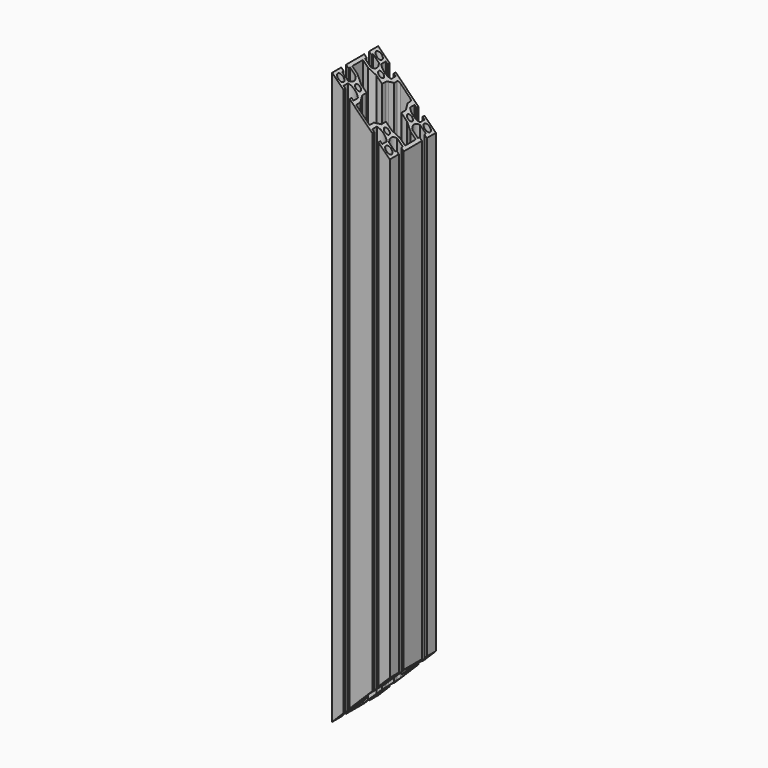
from build123d import *

# Parameters (mm, degrees)
F0_R     = 3
F0_R_2   = 2.5
F1_DEPTH = 595
F2_R     = 2
F3_R     = 7
F5_DEPTH = 60


# Not quite as in the source:
# - a feature names something its author has since deleted; it is built from what else it names


with BuildPart() as f1:
    # F0 (on Top) → F1 (new body)
    with BuildSketch(Plane.XY):
        with BuildLine():
            Line((18.15, -30), (30, -30))
            Line((30, -30), (30, -18.15))
            Line((30, -18.15), (27.5, -18.15))
            Line((27.5, -18.15), (27.5, -20.15))
            Line((27.5, -20.15), (21.5477069044, -20.15))
            ThreePointArc((21.5477069044, -20.15), (19.5, -15), (21.5477069044, -9.85))
            Line((21.5477069044, -9.85), (27.5, -9.85))
            Line((27.5, -9.85), (27.5, -11.85))
            Line((27.5, -11.85), (30, -11.85))
            Line((30, -11.85), (30, 11.85))
            Line((30, 11.85), (27.5, 11.85))
            Line((27.5, 11.85), (27.5, 9.85))
            Line((27.5, 9.85), (21.5477069044, 9.85))
            ThreePointArc((21.5477069044, 9.85), (19.5, 15), (21.5477069044, 20.15))
            Line((21.5477069044, 20.15), (27.5, 20.15))
            Line((27.5, 20.15), (27.5, 18.15))
            Line((27.5, 18.15), (30, 18.15))
            Line((30, 18.15), (30, 30))
            Line((30, 30), (18.15, 30))
            Line((18.15, 30), (18.15, 27.5))
            Line((18.15, 27.5), (20.15, 27.5))
            Line((20.15, 27.5), (20.15, 21.5477069044))
            ThreePointArc((20.15, 21.5477069044), (15, 19.5), (9.85, 21.5477069044))
            Line((9.85, 21.5477069044), (9.85, 27.5))
            Line((9.85, 27.5), (11.85, 27.5))
            Line((11.85, 27.5), (11.85, 30))
            Line((11.85, 30), (-11.85, 30))
            Line((-11.85, 30), (-11.85, 27.5))
            Line((-11.85, 27.5), (-9.85, 27.5))
            Line((-9.85, 27.5), (-9.85, 21.5477069044))
            ThreePointArc((-9.85, 21.5477069044), (-15, 19.5), (-20.15, 21.5477069044))
            Line((-20.15, 21.5477069044), (-20.15, 27.5))
            Line((-20.15, 27.5), (-18.15, 27.5))
            Line((-18.15, 27.5), (-18.15, 30))
            Line((-18.15, 30), (-30, 30))
            Line((-30, 30), (-30, 18.15))
            Line((-30, 18.15), (-27.5, 18.15))
            Line((-27.5, 18.15), (-27.5, 20.15))
            Line((-27.5, 20.15), (-21.5477069044, 20.15))
            ThreePointArc((-21.5477069044, 20.15), (-19.5, 15), (-21.5477069044, 9.85))
            Line((-21.5477069044, 9.85), (-27.5, 9.85))
            Line((-27.5, 9.85), (-27.5, 11.85))
            Line((-27.5, 11.85), (-30, 11.85))
            Line((-30, 11.85), (-30, -11.85))
            Line((-30, -11.85), (-27.5, -11.85))
            Line((-27.5, -11.85), (-27.5, -9.85))
            Line((-27.5, -9.85), (-21.5477069044, -9.85))
            ThreePointArc((-21.5477069044, -9.85), (-19.5, -15), (-21.5477069044, -20.15))
            Line((-21.5477069044, -20.15), (-27.5, -20.15))
            Line((-27.5, -20.15), (-27.5, -18.15))
            Line((-27.5, -18.15), (-30, -18.15))
            Line((-30, -18.15), (-30, -30))
            Line((-30, -30), (-18.15, -30))
            Line((-18.15, -30), (-18.15, -27.5))
            Line((-18.15, -27.5), (-20.15, -27.5))
            Line((-20.15, -27.5), (-20.15, -21.5477069044))
            ThreePointArc((-20.15, -21.5477069044), (-15, -19.5), (-9.85, -21.5477069044))
            Line((-9.85, -21.5477069044), (-9.85, -27.5))
            Line((-9.85, -27.5), (-11.85, -27.5))
            Line((-11.85, -27.5), (-11.85, -30))
            Line((-11.85, -30), (11.85, -30))
            Line((11.85, -30), (11.85, -27.5))
            Line((11.85, -27.5), (9.85, -27.5))
            Line((9.85, -27.5), (9.85, -21.5477069044))
            ThreePointArc((9.85, -21.5477069044), (15, -19.5), (20.15, -21.5477069044))
            Line((20.15, -21.5477069044), (20.15, -27.5))
            Line((20.15, -27.5), (18.15, -27.5))
            Line((18.15, -27.5), (18.15, -30))
        make_face()
        with Locations((-25, -25)):
            Circle(F0_R, mode=Mode.SUBTRACT)
        with Locations((-15, -15)):
            Circle(F0_R_2, mode=Mode.SUBTRACT)
        with Locations((25, -25)):
            Circle(F0_R, mode=Mode.SUBTRACT)
        with Locations((15, -15)):
            Circle(F0_R_2, mode=Mode.SUBTRACT)
        with Locations((-25, 25)):
            Circle(F0_R, mode=Mode.SUBTRACT)
        with Locations((-15, 15)):
            Circle(F0_R_2, mode=Mode.SUBTRACT)
        Polygon((-7, 22), (-7, 27.5), (0, 27.5), (7, 27.5), (7, 22), (10, 16), (10, 10), (16, 10), (22, 7), (27.5, 7), (27.5, 0), (27.5, -7), (22, -7), (16, -10), (10, -10), (10, -16), (7, -22), (7, -27.5), (0, -27.5), (-7, -27.5), (-7, -22), (-10, -16), (-10, -10), (-16, -10), (-22, -7), (-27.5, -7), (-27.5, 0), (-27.5, 7), (-22, 7), (-16, 10), (-10, 10), (-10, 16), align=None, mode=Mode.SUBTRACT)
        with Locations((15, 15)):
            Circle(F0_R_2, mode=Mode.SUBTRACT)
        with Locations((25, 25)):
            Circle(F0_R, mode=Mode.SUBTRACT)
    extrude(amount=F1_DEPTH)

    # F2
    f2_edges = [f1.edges().sort_by_distance(p)[0] for p in [
        (-7, 27.5, 297.5),
        (7, 27.5, 297.5),
    ]]
    fillet(f2_edges, radius=F2_R)

    # F3
    f3_edges = [f1.edges().sort_by_distance(p)[0] for p in [
        (-10, 16, 297.5),
        (10, 16, 297.5),
    ]]
    fillet(f3_edges, radius=F3_R)

    # F4 (on face) → F5 (cut)
    with BuildSketch(Plane.XZ.offset(30)):
        Polygon((30, 0), (30, 60), (-30, 0), (-18.15, 0), align=None)
        Polygon((30, 535), (30, 595), (-18.15, 595), (-30, 595), align=None)
    extrude(amount=-F5_DEPTH, mode=Mode.SUBTRACT)


solid = f1.part
